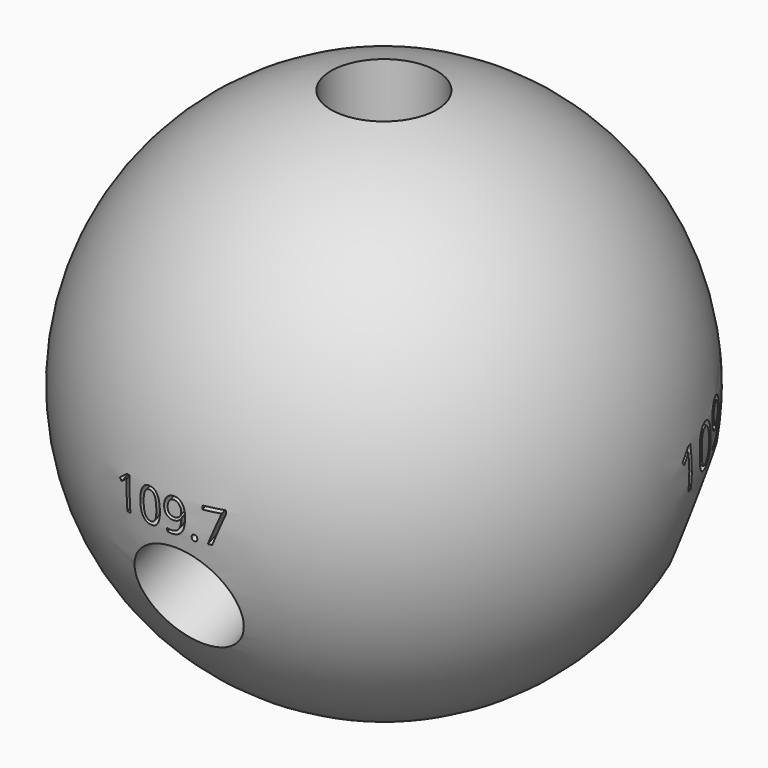
from build123d import *

# Parameters (mm, degrees)
F3_R          = 3.175
F4_DEPTH      = 25.4
F7_ANGLE      = 109.7
F8_ANGLE      = 108
F9_ANGLE      = 30
F11_TEXT_SIZE = 2.6826691788
F12_DEPTH     = 6.35
F14_TEXT_SIZE = 2.8036424838
F15_DEPTH     = 6.35
F16_ANGLE     = 109.4
F17_ANGLE     = -30
F19_TEXT_SIZE = 3.5347384659
F20_DEPTH     = 6.35


# Not quite as in the source:
# - Text() gives the source's letters only with a copy of the font that has no kerning and outlines rounded to 1/6400 em; it was checked with that copy


with BuildPart() as f1:
    # F0 (on Front) → F1 (revolve)
    with BuildSketch(Plane.XZ):
        with BuildLine():
            Line((0, -15.875), (0, 15.875))
            ThreePointArc((0, 15.875), (-15.875, 0), (0, -15.875))
        make_face()
    revolve(axis=Axis((0, 0, 0), (0, 0, -1)))

    # F11 (on offset) → F12 (cut)
    with BuildSketch(Plane(origin=(0, -17.5613677562, -6.2878799923), x_dir=(1, 0, 0), z_dir=(0, -0.9414705448, -0.3370952584))):
        with Locations((-3.7342637661, 3.9106665645)):
            Text('109.7', F11_TEXT_SIZE, font='Open Sans', text_align=(TextAlign.LEFT, TextAlign.BOTTOM))
    extrude(amount=-F12_DEPTH, mode=Mode.SUBTRACT)

    # F14 (on offset) → F15 (cut)
    with BuildSketch(Plane(origin=(-15.3634431533, 8.8700880403, -5.7641326232), x_dir=(-0.4452239052, -0.8797004466, -0.1670413078), z_dir=(-0.8236391035, 0.4755282581, -0.3090169944))):
        with Locations((-2.4227413683, 4.0223049)):
            Text('108', F14_TEXT_SIZE, font='Open Sans', text_align=(TextAlign.LEFT, TextAlign.BOTTOM))
    extrude(amount=-F15_DEPTH, mode=Mode.SUBTRACT)

    # F19 (on offset) → F20 (cut)
    with BuildSketch(Plane(origin=(15.236894378, 8.7970250708, -6.1958431132), x_dir=(-0.436873574, 0.8818065289, 0.177647758), z_dir=(0.8168547832, 0.471611329, -0.3321611319))):
        with Locations((-4.5912938855, 3.5619535483)):
            Text('109.4', F19_TEXT_SIZE, font='Open Sans', text_align=(TextAlign.LEFT, TextAlign.BOTTOM))
    extrude(amount=-F20_DEPTH, mode=Mode.SUBTRACT)


with BuildPart() as f4:
    # F3 (on offset) → F4 (new body)
    with BuildSketch(Plane.XY.offset(5.953125)):
        Circle(F3_R)
    extrude(amount=F4_DEPTH)


with BuildPart() as f7_1:
    # F7: copy of F4
    add(f4.part.rotate(Axis((-9.2145558447, 0, 0), (1, 0, 0)), F7_ANGLE))


with BuildPart() as f8_1:
    # F8: copy of F4
    add(f4.part.rotate(Axis((0, 1.4487542212, 0), (0, -1, 0)), F8_ANGLE))


with BuildPart() as f8_1_1:
    # F9: moved
    add(f8_1.part.rotate(Axis((0, 0, 3.344045952), (0, 0, -1)), F9_ANGLE))


with BuildPart() as f16_1:
    # F16: copy of F4
    add(f4.part.rotate(Axis((0, 26.1310953647, 0), (0, 1, 0)), F16_ANGLE))


with BuildPart() as f16_1_1:
    # F17: moved
    add(f16_1.part.rotate(Axis((0, 0, 3.344045952), (0, 0, -1)), F17_ANGLE))


with BuildPart() as f1_1:
    add(f1.part)

    # F21: cut F7_1, F8_1, F16_1, F4
    add(f7_1.part, mode=Mode.SUBTRACT)
    add(f8_1_1.part, mode=Mode.SUBTRACT)
    add(f16_1_1.part, mode=Mode.SUBTRACT)
    add(f4.part, mode=Mode.SUBTRACT)


solid = f1_1.part
